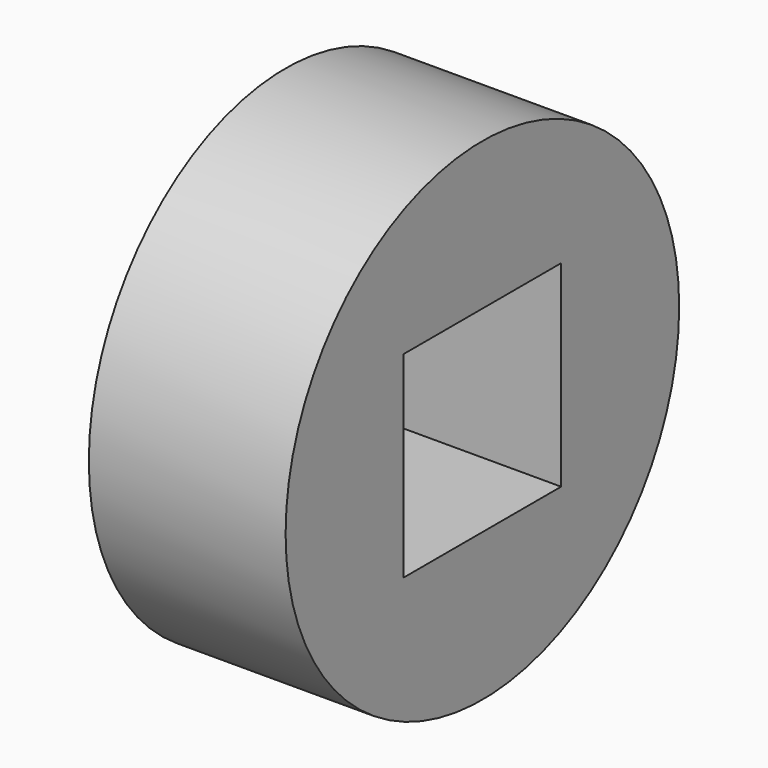
from build123d import *

# Parameters (mm, degrees)
F0_R          = 12.5
F2_DEPTH      = 5
F1_W          = 10
F1_H          = 10
F3_DEPTH      = 5.001
F3_DEPTH_BACK = 5.001


with BuildPart() as f2:
    # F0 (on Right) → F2 (new body, symmetric)
    with BuildSketch(Plane.YZ):
        Circle(F0_R)
    extrude(amount=F2_DEPTH, both=True)

    # F1 (on Right) → F3 (cut, two sides)
    with BuildSketch(Plane.YZ) as f3_sk:
        Rectangle(F1_W, F1_H)
    extrude(amount=-F3_DEPTH, mode=Mode.SUBTRACT)
    extrude(f3_sk.sketch, amount=F3_DEPTH_BACK, mode=Mode.SUBTRACT)


solid = f2.part
